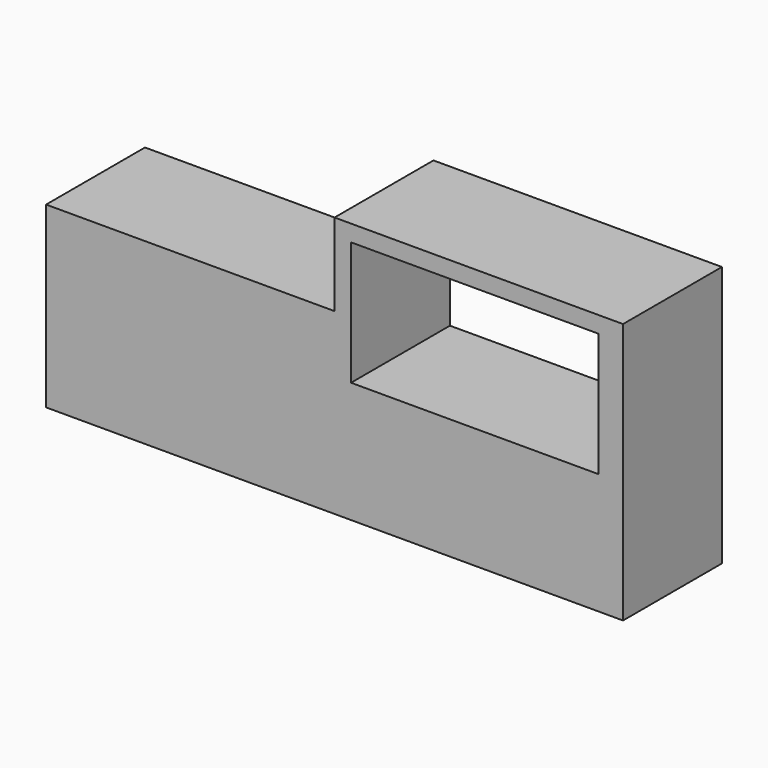
from build123d import *

# Parameters (mm, degrees)
F1_DEPTH = 457.2
F2_W     = 914.4
F2_H     = 457.2
F3_DEPTH = 457.2
F4_T     = -60.96


# Not quite as in the source:
# - a shell that OpenCascade refuses in one call is made with other operations: the cavity is built on its own and cut out


with BuildPart() as f1:
    # F0 (on Front) → F1 (new body)
    with BuildSketch(Plane.XZ):
        Polygon((-0.0530799283, 304.7990856), (-0.0530799283, 0), (-1066.8530799283, 0), (-1066.8530799283, -660.401016), (-0.0530799283, -660.401016), (1066.7469200717, -660.401016), (1066.7469200717, 304.7990856), align=None)
    extrude(amount=-F1_DEPTH)

    # F2 (on face) → F3 (cut, through all)
    with BuildSketch(Plane.XZ):
        with Locations((518.1069200717, 15.2390856)):
            Rectangle(F2_W, F2_H)
    extrude(amount=-F3_DEPTH, mode=Mode.SUBTRACT)

    # F4: a shell. OpenCascade refuses it in one call, so the cavity is built on its own and cut out:
    # the body offset inwards by the wall thickness, plus a prism from it out through each open face.
    f4_core = offset(f1.part, amount=F4_T, kind=Kind.INTERSECTION, mode=Mode.PRIVATE)
    f4_exits = [f4_core.faces().sort_by_distance(p)[0] for p in [
        (-124.304275, 396.24, -370.362523),
    ]]
    add(f4_core, mode=Mode.SUBTRACT)
    extrude(f4_exits, amount=-F4_T, mode=Mode.SUBTRACT)


solid = f1.part
